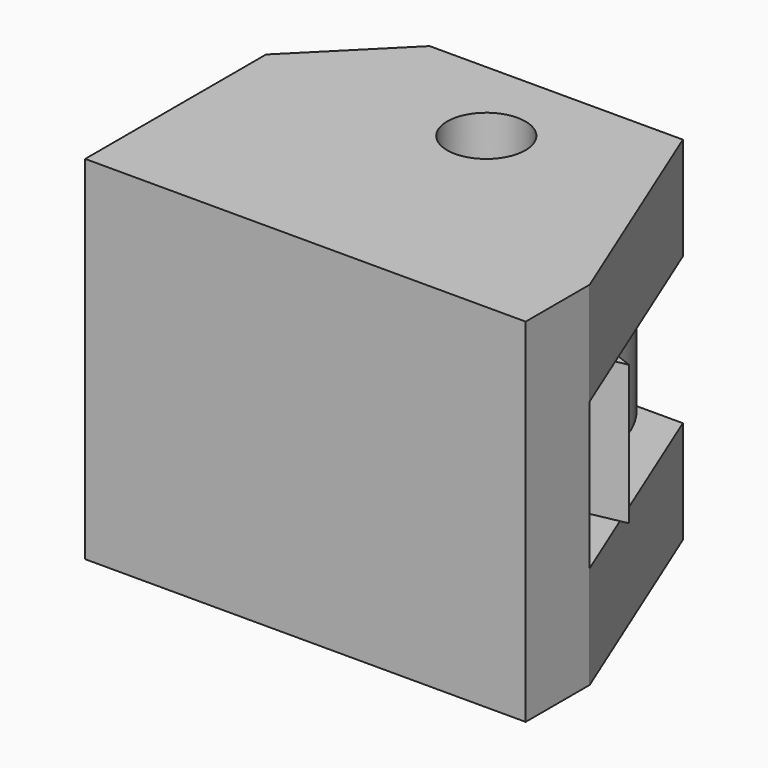
from build123d import *

# Parameters (mm, degrees)
F1_R      = 4.2
F1_R_2    = 2.665
F3_DEPTH  = 7
F5_R      = 2.665
F6_DEPTH  = 7
F2_R      = 1.625
F7_DEPTH  = 9.5
F10_DEPTH = 10


# Not quite as in the source:
# - the program builds the solid bodies; features that only make, move or delete a surface that nothing else refers to are left out


with BuildPart() as f3:
    # F1 (on Top) → F3 (new body)
    with BuildSketch(Plane.XY):
        Polygon((-8.8110024968, 6.1889975032), (-15, 0), (-15, -15.3994522989), (15, -15.3994522989), (15, -9.9498743711), (8.4334993606, 6.1889975032), align=None)
        Circle(F1_R, mode=Mode.SUBTRACT)
        Circle(F1_R)
        Circle(F1_R_2, mode=Mode.SUBTRACT)
    extrude(amount=F3_DEPTH)



with BuildPart() as f6:
    # F5 (on offset) → F6 (new body)
    with BuildSketch(Plane(origin=(0, 0, -10), x_dir=(1, 0, 0), z_dir=(0, 0, -1))):
        Polygon((-15, 0), (-8.8110024968, -6.1889975032), (8.4334993606, -6.1889975032), (15, 9.9498743711), (15, 15.3994522989), (-15, 15.3994522989), align=None)
        Circle(F5_R, mode=Mode.SUBTRACT)
    extrude(amount=F6_DEPTH)


with BuildPart() as f7:
    # F2 (on Top) → F7 (new body)
    with BuildSketch(Plane.XY):
        with BuildLine():
            Line((1.5724151216, -7.8439473918), (14.0134819596, -5.3499834923))
            Line((14.0134819596, -5.3499834923), (11.2107855677, -4.2799867939))
            ThreePointArc((11.2107855677, -4.2799867939), (8.919201221, -2.5062544394), (7.996377476, 0.240722375))
            ThreePointArc((7.996377476, 0.240722375), (-6.2634590486, 4.9768545033), (1.5724151216, -7.8439473918))
        make_face()
        Circle(F2_R, mode=Mode.SUBTRACT)
    extrude(amount=-F7_DEPTH)


with BuildPart() as f3_1:
    add(f3.part)

    add(f6.part)  # F10 merges F6
    # F9 (on face) → F10 (join, through all)
    with BuildSketch(Plane.XY.offset(-10)):
        with BuildLine():
            Line((-9.351134908, -3.3994522989), (-15, -3.3994522989))
            Line((-15, -3.3994522989), (-15, -15.3994522989))
            Line((-15, -15.3994522989), (15, -15.3994522989))
            Line((15, -15.3994522989), (15, -9.9498743711))
            Line((15, -9.9498743711), (0, -9.9498743711))
            ThreePointArc((0, -9.9498743711), (-5.7085846186, -8.1493595854), (-9.351134908, -3.3994522989))
        make_face()
    extrude(amount=F10_DEPTH)


solid = Compound([f7.part, f3_1.part])
